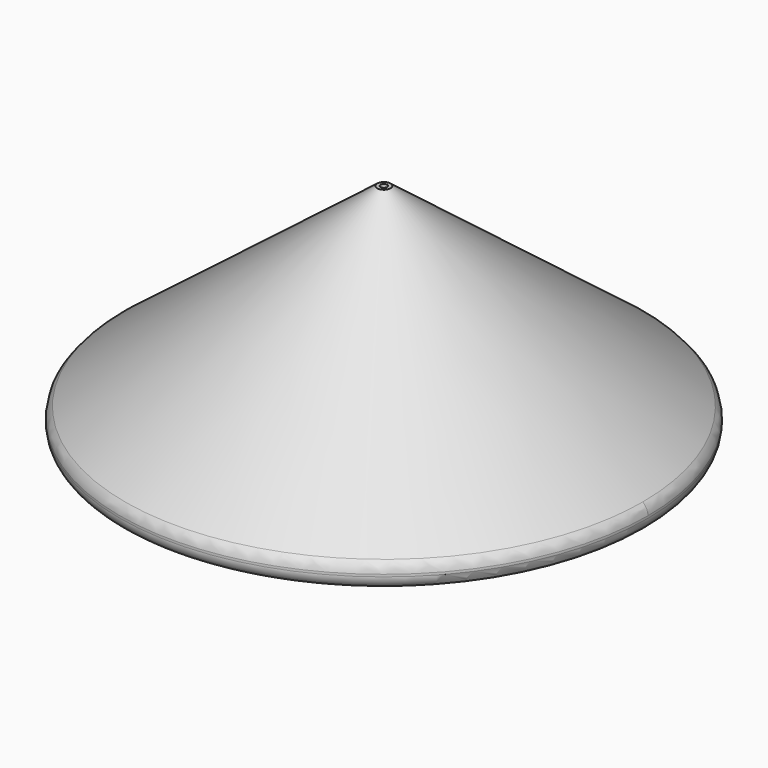
from build123d import *

# Parameters (mm, degrees)
F0_R      = 60
F0_R_2    = 40
F3_DEPTH  = 3
F4_R      = 60
F4_R_2    = 40
F5_DEPTH  = 2
F9_R      = 3
F10_R     = 0.75
F11_DEPTH = 50.001


# Not quite as in the source:
# - a fillet or chamfer that OpenCascade refuses, or shapes differently, is made with other operations: its cross-section is extruded or revolved along the edge and cut away or added


with BuildPart() as f3:
    # F0 (on Top) → F3 (new body)
    with BuildSketch(Plane.XY):
        Circle(F0_R)
        Polygon((-25, -34.4095480118), (-25, -42.9095480118), (-31.175611488, -42.9095480118), (-33.0839803885, -37.036192464), align=None, mode=Mode.SUBTRACT)
        Polygon((25, -34.4095480118), (33.0839803885, -37.036192464), (31.175611488, -42.9095480118), (25, -42.9095480118), align=None, mode=Mode.SUBTRACT)
        Polygon((-45.4470243632, 20.0199222552), (-40.4508497187, 13.143277803), (-48.5348301073, 10.5166333508), (-50.4431990077, 16.3899888986), align=None, mode=Mode.SUBTRACT)
        Circle(F0_R_2, mode=Mode.SUBTRACT)
        Polygon((50.4431990077, 16.3899888986), (48.5348301073, 10.5166333508), (40.4508497187, 13.143277803), (45.4470243632, 20.0199222552), align=None, mode=Mode.SUBTRACT)
        Polygon((4.9961746445, 49.4091848698), (0, 42.5325404176), (-4.9961746445, 49.4091848698), (0, 53.0391182264), align=None, mode=Mode.SUBTRACT)
    extrude(amount=F3_DEPTH)

    # F4 (on face) → F5 (join)
    with BuildSketch(Plane.XY.offset(3)):
        Circle(F4_R)
        Polygon((-31.175611488, -42.9095480118), (-33.0839803885, -37.036192464), (-25, -34.4095480118), (-25, -42.9095480118), align=None, mode=Mode.SUBTRACT)
        Polygon((25, -42.9095480118), (25, -34.4095480118), (33.0839803885, -37.036192464), (31.175611488, -42.9095480118), align=None, mode=Mode.SUBTRACT)
        Polygon((-40.4508497187, 13.143277803), (-48.5348301073, 10.5166333508), (-50.4431990077, 16.3899888986), (-45.4470243632, 20.0199222552), align=None, mode=Mode.SUBTRACT)
        Circle(F4_R_2, mode=Mode.SUBTRACT)
        Polygon((40.4508497187, 13.143277803), (45.4470243632, 20.0199222552), (50.4431990077, 16.3899888986), (48.5348301073, 10.5166333508), align=None, mode=Mode.SUBTRACT)
        Polygon((0, 53.0391182264), (4.9961746445, 49.4091848698), (0, 42.5325404176), (-4.9961746445, 49.4091848698), align=None, mode=Mode.SUBTRACT)
        Polygon((-50.4431990077, 16.3899888986), (-48.5348301073, 10.5166333508), (-40.4508497187, 13.143277803), (-45.4470243632, 20.0199222552), align=None)
        Polygon((0, 42.5325404176), (4.9961746445, 49.4091848698), (0, 53.0391182264), (-4.9961746445, 49.4091848698), align=None)
        Polygon((50.4431990077, 16.3899888986), (45.4470243632, 20.0199222552), (40.4508497187, 13.143277803), (48.5348301073, 10.5166333508), align=None)
        Polygon((33.0839803885, -37.036192464), (25, -34.4095480118), (25, -42.9095480118), (31.175611488, -42.9095480118), align=None)
        Polygon((-25, -34.4095480118), (-33.0839803885, -37.036192464), (-31.175611488, -42.9095480118), (-25, -42.9095480118), align=None)
    extrude(amount=F5_DEPTH)

    # F6 (on Front) → F8 (revolve)
    with BuildSketch(Plane.XZ):
        Polygon((-1.5, 50), (-60, 5), (-40.3058288648, 5), (0, 47), (0, 50), align=None)
    revolve(axis=Axis((0, 0, 19.0761145204), (0, 0, 1)))

    # F9
    f9_edges = [f3.edges().sort_by_distance(p)[0] for p in [
        (0, -60, 5),
        (0, 60, 5),
        (-60, 0, 0),
    ]]
    fillet(f9_edges, radius=F9_R)

    # F10 (on offset) → F11 (cut, through all)
    with BuildSketch(Plane.XY.offset(50)):
        Circle(F10_R)
    extrude(amount=-F11_DEPTH, mode=Mode.SUBTRACT)

    # F12: fillet of radius 5 on 1 edges, made by hand

    # F12_s1 → F12_t2 (revolve, cut)
    with BuildSketch(Plane.XZ):
        with BuildLine():
            ThreePointArc((40, 3.2781529238), (40.0770509003, 4.1525510952), (40.3058288648, 5))
            Line((40.3058288648, 5), (40.2119454421, 5.0344369415))
            ThreePointArc((40.2119454421, 5.0344369415), (40.1529144324, 5.1), (40, 5.1))
            Line((40, 5.1), (39.9, 5))
            Line((39.9, 5), (39.9, 3.2781529238))
            Line((39.9, 3.2781529238), (40, 3.2781529238))
        make_face()
    revolve(axis=Axis((0, 0, 5), (0, 0, 1)), mode=Mode.SUBTRACT)


solid = f3.part
